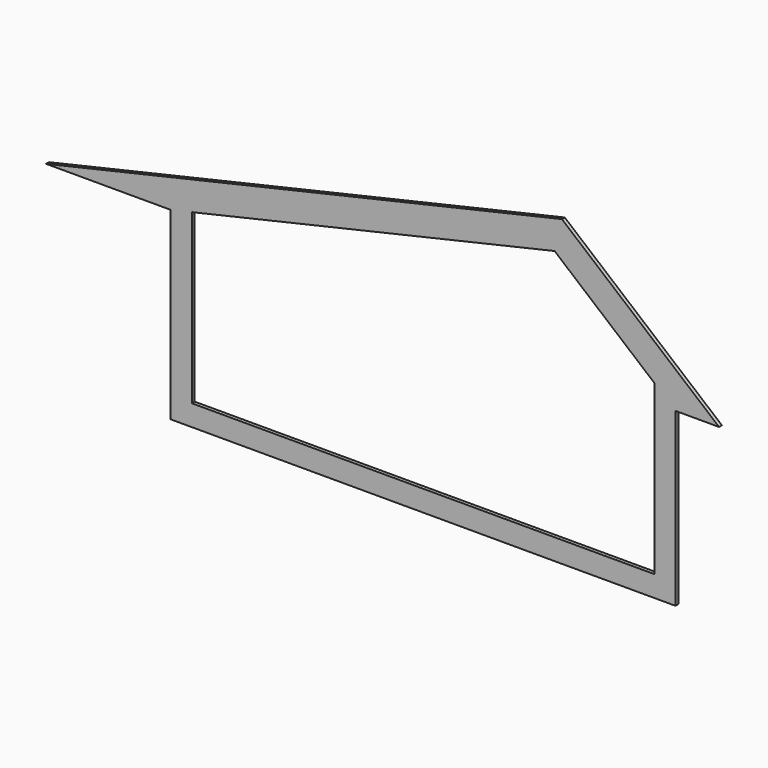
from build123d import *

# Parameters (mm, degrees)
F1_DEPTH = 51


# Not quite as in the source:
# - a feature of the source that left no trace in its solid (it failed there, or was rolled back) is left out
# - a feature names something its author has since deleted; it is built from what else it names


with BuildPart() as f1:
    # F0 (on Front) → F1 (new body)
    with BuildSketch(Plane.XZ):
        Polygon((6900, 2400), (6900, 0), (7200, 0), (7200, 2148.2701106468), align=None)
        Polygon((-1778.1645930343, 2330.7395426623), (0, 2330.7395426623), (300, 2400), (5475.9103875206, 3594.9530685949), (6900, 2400), (7200, 2148.2701106468), (7822.2895307442, 2148.2701106468), (5580.2511632789, 4029.5636778722), align=None)
        Polygon((300, 0), (0, 0), (0, -300), (7200, -300), (7200, 0), (6900, 0), align=None)
        Polygon((0, 2330.7395426623), (0, 0), (300, 0), (300, 2400), align=None)
    extrude(amount=F1_DEPTH)


solid = f1.part
